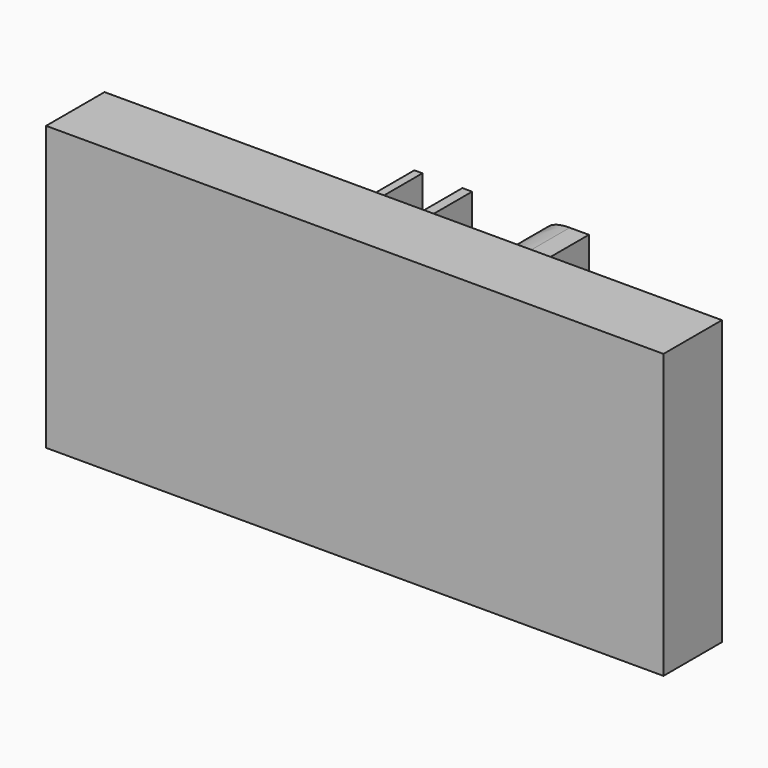
from build123d import *

# Parameters (mm, degrees)
F1_DEPTH     = 20
F2_TEXT_SIZE = 28.3416975031
F3_DEPTH     = 50


# Not quite as in the source:
# - Text() gives the source's letters only with a copy of the font that has no kerning and outlines rounded to 1/6400 em; it was checked with that copy


with BuildPart() as f1:
    # F0 (on Front) → F1 (new body)
    with BuildSketch(Plane.XZ):
        with BuildLine():
            Line((126.0287463665, 41.8179742992), (-42.9676100612, 41.8179742992))
            Line((-42.9676100612, 41.8179742992), (-42.9676100612, -34.1471293349))
            add(Edge.make_bspline(
                [(-42.9676100612, -35.7823930681), (-42.5012247819, -35.3164509597), (-42.5519245801, -34.7172980233), (-42.9676100612, -34.1471293349)],
                knots=[0, 0, 0, 0, 0.1042973693, 0.1042973693, 0.1042973693, 0.1042973693], degree=3))
            Line((-42.9676100612, -35.7823930681), (126.0287463665, -35.7823930681))
            Line((126.0287463665, -35.7823930681), (126.0287463665, 41.8179742992))
        make_face()
        with BuildLine():
            add(Edge.make_bspline(
                [(-42.9676100612, -35.7823930681), (-42.5012247819, -35.3164509597), (-42.5519245801, -34.7172980233), (-42.9676100612, -34.1471293349)],
                knots=[0, 0, 0, 0, 0.1042973693, 0.1042973693, 0.1042973693, 0.1042973693], degree=3))
            Line((-42.9676100612, -34.1471293349), (-42.9676100612, -35.7823930681))
        make_face()
    extrude(amount=F1_DEPTH)

    # F2 (on face) → F3 (join)
    with BuildSketch(Plane(origin=(0, 0, 0), x_dir=(-1, 0, 0), z_dir=(0, 1, 0))):
        with Locations((-52.3922848686, -3.0177920125)):
            Text('P. N', F2_TEXT_SIZE, font='Open Sans', text_align=(TextAlign.LEFT, TextAlign.BOTTOM))
    extrude(amount=F3_DEPTH)


solid = f1.part
